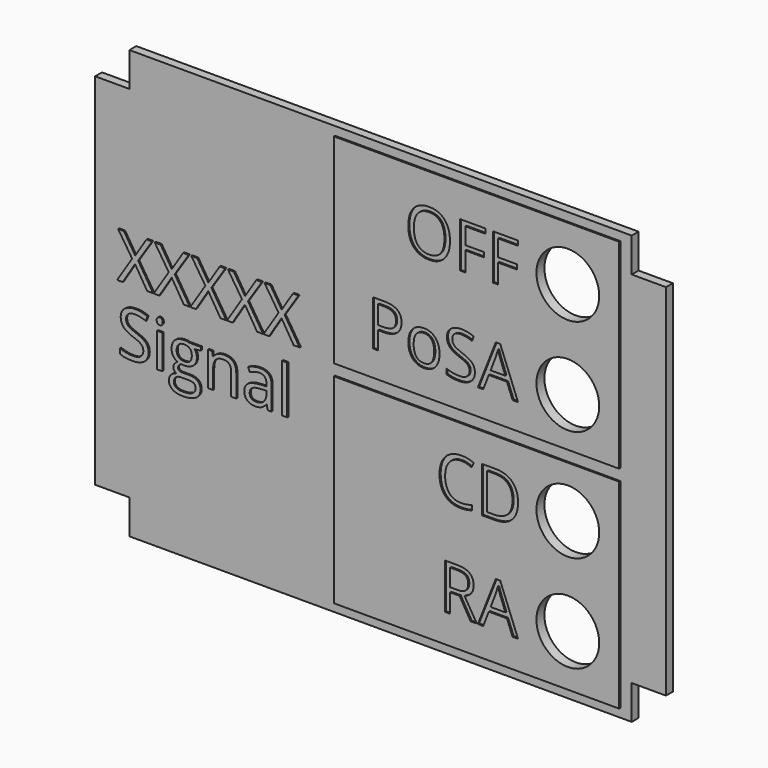
from build123d import *

# Parameters (mm, degrees)
F0_R         = 11
F1_DEPTH     = 3
F2_W         = 100
F2_H         = 70
F2_R         = 11
F2_TEXT_SIZE = 22.2222222222
F3_DEPTH     = 0.5


# Not quite as in the source:
# - Text() gives the source's letters only with a copy of the font that has no kerning and outlines rounded to 1/6400 em; it was checked with that copy


with BuildPart() as f1:
    # F0 (on Front) → F1 (new body)
    with BuildSketch(Plane.XZ):
        Polygon((35.0830127597, 118.6418436468), (-140.9169872403, 118.6418436468), (-140.9169872403, 106.6418436468), (-152.9169872403, 106.6418436468), (-152.9169872403, -19.3581563532), (-140.9169872403, -19.3581563532), (-140.9169872403, -31.3581563532), (35.0830127597, -31.3581563532), (35.0830127597, -19.3581563532), (47.0830127597, -19.3581563532), (47.0830127597, 106.6418436468), (35.0830127597, 106.6418436468), align=None)
        with Locations((13.0830127597, -10.3581563532)):
            Circle(F0_R, mode=Mode.SUBTRACT)
        with Locations((13.0830127597, 23.6418436468)):
            Circle(F0_R, mode=Mode.SUBTRACT)
        with Locations((13.0830127597, 62.6418436468)):
            Circle(F0_R, mode=Mode.SUBTRACT)
        with Locations((13.0830127597, 96.6418436468)):
            Circle(F0_R, mode=Mode.SUBTRACT)
    extrude(amount=F1_DEPTH)

    # F2 (on face) → F3 (join)
    with BuildSketch(Plane.XZ.offset(3)):
        with Locations((-18.9169872403, 6.6418436468)):
            Rectangle(F2_W, F2_H)
        with BuildLine():
            Line((-24.8197650181, -11.760934131), (-28.1322650181, -11.760934131))
            Line((-28.1322650181, -11.760934131), (-28.1322650181, -18.3581563532))
            Line((-28.1322650181, -18.3581563532), (-29.9760150181, -18.3581563532))
            Line((-29.9760150181, -18.3581563532), (-29.9760150181, -2.4935730199))
            Line((-29.9760150181, -2.4935730199), (-25.6253205736, -2.4935730199))
            add(Edge.make_bspline(
                [(-25.6253205736, -2.4935730199), (-22.7051816848, -2.4935730199), (-21.3110844625, -3.6116285755)],
                knots=[0, 0, 0, 1, 1, 1], degree=2))
            add(Edge.make_bspline(
                [(-21.3110844625, -3.6116285755), (-19.9169872403, -4.729684131), (-19.9169872403, -6.9762119088)],
                knots=[0, 0, 0, 1, 1, 1], degree=2))
            add(Edge.make_bspline(
                [(-19.9169872403, -6.9762119088), (-19.9169872403, -10.1220452421), (-23.1079594625, -11.229684131)],
                knots=[0, 0, 0, 1, 1, 1], degree=2))
            Line((-23.1079594625, -11.229684131), (-18.7989316848, -18.3581563532))
            Line((-18.7989316848, -18.3581563532), (-20.9794872403, -18.3581563532))
            Line((-20.9794872403, -18.3581563532), (-24.8197650181, -11.760934131))
        make_face(mode=Mode.SUBTRACT)
        Polygon((-4.3579594625, -18.3581563532), (-6.2676816848, -18.3581563532), (-8.2433761292, -13.3130174643), (-14.6010150181, -13.3130174643), (-16.552403907, -18.3581563532), (-18.4204594625, -18.3581563532), (-12.1496261292, -2.4276007977), (-10.5975427959, -2.4276007977), align=None, mode=Mode.SUBTRACT)
        with Locations((13.0830127597, -10.3581563532)):
            Circle(F2_R, mode=Mode.SUBTRACT)
        with BuildLine():
            add(Edge.make_bspline(
                [(-20.646153907, 29.239065869), (-22.4482372403, 30.082815869), (-24.2503205736, 30.082815869)],
                knots=[0, 0, 0, 1, 1, 1], degree=2))
            add(Edge.make_bspline(
                [(-24.2503205736, 30.082815869), (-26.864903907, 30.082815869), (-28.3787927959, 28.3414964245)],
                knots=[0, 0, 0, 1, 1, 1], degree=2))
            add(Edge.make_bspline(
                [(-28.3787927959, 28.3414964245), (-29.8926816848, 26.6001769801), (-29.8926816848, 23.5723992023)],
                knots=[0, 0, 0, 1, 1, 1], degree=2))
            add(Edge.make_bspline(
                [(-29.8926816848, 23.5723992023), (-29.8926816848, 20.4612880912), (-28.4326122403, 18.7616353134)],
                knots=[0, 0, 0, 1, 1, 1], degree=2))
            add(Edge.make_bspline(
                [(-28.4326122403, 18.7616353134), (-26.9725427959, 17.0619825357), (-24.271153907, 17.0619825357)],
                knots=[0, 0, 0, 1, 1, 1], degree=2))
            add(Edge.make_bspline(
                [(-24.271153907, 17.0619825357), (-22.6114316848, 17.0619825357), (-20.4829594625, 17.6592047579)],
                knots=[0, 0, 0, 1, 1, 1], degree=2))
            Line((-20.4829594625, 17.6592047579), (-20.4829594625, 16.0446214245))
            add(Edge.make_bspline(
                [(-20.4829594625, 16.0446214245), (-22.1322650181, 15.4230936468), (-24.552403907, 15.4230936468)],
                knots=[0, 0, 0, 1, 1, 1], degree=2))
            add(Edge.make_bspline(
                [(-24.552403907, 15.4230936468), (-28.0558761292, 15.4230936468), (-29.9603900181, 17.551565869)],
                knots=[0, 0, 0, 1, 1, 1], degree=2))
            add(Edge.make_bspline(
                [(-29.9603900181, 17.551565869), (-31.864903907, 19.6800380912), (-31.864903907, 23.5967047579)],
                knots=[0, 0, 0, 1, 1, 1], degree=2))
            add(Edge.make_bspline(
                [(-31.864903907, 23.5967047579), (-31.864903907, 26.0480936468), (-30.9482372403, 27.8918436468)],
                knots=[0, 0, 0, 1, 1, 1], degree=2))
            add(Edge.make_bspline(
                [(-30.9482372403, 27.8918436468), (-30.0315705736, 29.7355936468), (-28.3006677959, 30.7338575357)],
                knots=[0, 0, 0, 1, 1, 1], degree=2))
            add(Edge.make_bspline(
                [(-28.3006677959, 30.7338575357), (-26.5697650181, 31.7321214245), (-24.2260150181, 31.7321214245)],
                knots=[0, 0, 0, 1, 1, 1], degree=2))
            add(Edge.make_bspline(
                [(-24.2260150181, 31.7321214245), (-21.7329594625, 31.7321214245), (-19.864903907, 30.8223992023)],
                knots=[0, 0, 0, 1, 1, 1], degree=2))
            Line((-19.864903907, 30.8223992023), (-20.646153907, 29.239065869))
        make_face(mode=Mode.SUBTRACT)
        with BuildLine():
            add(Edge.make_bspline(
                [(-6.4083066848, 29.4560797579), (-4.3579594625, 27.4057325357), (-4.3579594625, 23.7251769801)],
                knots=[0, 0, 0, 1, 1, 1], degree=2))
            add(Edge.make_bspline(
                [(-4.3579594625, 23.7251769801), (-4.3579594625, 19.7980936468), (-6.489903907, 17.7199686468)],
                knots=[0, 0, 0, 1, 1, 1], degree=2))
            add(Edge.make_bspline(
                [(-6.489903907, 17.7199686468), (-8.6218483514, 15.6418436468), (-12.6253205736, 15.6418436468)],
                knots=[0, 0, 0, 1, 1, 1], degree=2))
            Line((-12.6253205736, 15.6418436468), (-17.021153907, 15.6418436468))
            Line((-17.021153907, 15.6418436468), (-17.021153907, 31.5064269801))
            Line((-17.021153907, 31.5064269801), (-12.1600427959, 31.5064269801))
            add(Edge.make_bspline(
                [(-12.1600427959, 31.5064269801), (-8.458653907, 31.5064269801), (-6.4083066848, 29.4560797579)],
                knots=[0, 0, 0, 1, 1, 1], degree=2))
        make_face(mode=Mode.SUBTRACT)
        with Locations((13.0830127597, 23.6418436468)):
            Circle(F2_R, mode=Mode.SUBTRACT)
        with Locations((-18.9169872403, 80.6418436468)):
            Rectangle(F2_W, F2_H)
        with BuildLine():
            add(Edge.make_bspline(
                [(-33.3388622403, 65.0914964245), (-31.8683761292, 63.4300380912), (-31.8683761292, 60.6001769801)],
                knots=[0, 0, 0, 1, 1, 1], degree=2))
            add(Edge.make_bspline(
                [(-31.8683761292, 60.6001769801), (-31.8683761292, 57.6904547579), (-33.3319177959, 56.0567742023)],
                knots=[0, 0, 0, 1, 1, 1], degree=2))
            add(Edge.make_bspline(
                [(-33.3319177959, 56.0567742023), (-34.7954594625, 54.4230936468), (-37.3787927959, 54.4230936468)],
                knots=[0, 0, 0, 1, 1, 1], degree=2))
            add(Edge.make_bspline(
                [(-37.3787927959, 54.4230936468), (-38.9760150181, 54.4230936468), (-40.2121261292, 55.1730936468)],
                knots=[0, 0, 0, 1, 1, 1], degree=2))
            add(Edge.make_bspline(
                [(-40.2121261292, 55.1730936468), (-41.4482372403, 55.9230936468), (-42.1218483514, 57.3223992023)],
                knots=[0, 0, 0, 1, 1, 1], degree=2))
            add(Edge.make_bspline(
                [(-42.1218483514, 57.3223992023), (-42.7954594625, 58.7217047579), (-42.7954594625, 60.6001769801)],
                knots=[0, 0, 0, 1, 1, 1], degree=2))
            add(Edge.make_bspline(
                [(-42.7954594625, 60.6001769801), (-42.7954594625, 63.5064269801), (-41.3405983514, 65.129690869)],
                knots=[0, 0, 0, 1, 1, 1], degree=2))
            add(Edge.make_bspline(
                [(-41.3405983514, 65.129690869), (-39.8857372403, 66.7529547579), (-37.302403907, 66.7529547579)],
                knots=[0, 0, 0, 1, 1, 1], degree=2))
            add(Edge.make_bspline(
                [(-37.302403907, 66.7529547579), (-34.8093483514, 66.7529547579), (-33.3388622403, 65.0914964245)],
                knots=[0, 0, 0, 1, 1, 1], degree=2))
        make_face(mode=Mode.SUBTRACT)
        with BuildLine():
            add(Edge.make_bspline(
                [(-51.1253205736, 70.5064269801), (-45.1808761292, 70.5064269801), (-45.1808761292, 65.8848992023)],
                knots=[0, 0, 0, 1, 1, 1], degree=2))
            add(Edge.make_bspline(
                [(-45.1808761292, 65.8848992023), (-45.1808761292, 63.4751769801), (-46.8249733514, 62.1783019801)],
                knots=[0, 0, 0, 1, 1, 1], degree=2))
            add(Edge.make_bspline(
                [(-46.8249733514, 62.1783019801), (-48.4690705736, 60.8814269801), (-51.5280983514, 60.8814269801)],
                knots=[0, 0, 0, 1, 1, 1], degree=2))
            Line((-51.5280983514, 60.8814269801), (-53.396153907, 60.8814269801))
            Line((-53.396153907, 60.8814269801), (-53.396153907, 54.6418436468))
            Line((-53.396153907, 54.6418436468), (-55.239903907, 54.6418436468))
            Line((-55.239903907, 54.6418436468), (-55.239903907, 70.5064269801))
            Line((-55.239903907, 70.5064269801), (-51.1253205736, 70.5064269801))
        make_face(mode=Mode.SUBTRACT)
        with BuildLine():
            add(Edge.make_bspline(
                [(-20.4239316848, 61.5098992023), (-19.4864316848, 60.489065869), (-19.4864316848, 58.864065869)],
                knots=[0, 0, 0, 1, 1, 1], degree=2))
            add(Edge.make_bspline(
                [(-19.4864316848, 58.864065869), (-19.4864316848, 56.770315869), (-21.005528907, 55.5967047579)],
                knots=[0, 0, 0, 1, 1, 1], degree=2))
            add(Edge.make_bspline(
                [(-21.005528907, 55.5967047579), (-22.5246261292, 54.4230936468), (-25.1287927959, 54.4230936468)],
                knots=[0, 0, 0, 1, 1, 1], degree=2))
            add(Edge.make_bspline(
                [(-25.1287927959, 54.4230936468), (-27.9482372403, 54.4230936468), (-29.4690705736, 55.1522603134)],
                knots=[0, 0, 0, 1, 1, 1], degree=2))
            Line((-29.4690705736, 55.1522603134), (-29.4690705736, 56.9300380912))
            add(Edge.make_bspline(
                [(-29.4690705736, 56.9300380912), (-28.489903907, 56.520315869), (-27.3405983514, 56.2807325357)],
                knots=[0, 0, 0, 1, 1, 1], degree=2))
            add(Edge.make_bspline(
                [(-27.3405983514, 56.2807325357), (-26.1912927959, 56.0411492023), (-25.0628205736, 56.0411492023)],
                knots=[0, 0, 0, 1, 1, 1], degree=2))
            add(Edge.make_bspline(
                [(-25.0628205736, 56.0411492023), (-23.2190705736, 56.0411492023), (-22.2850427959, 56.7408019801)],
                knots=[0, 0, 0, 1, 1, 1], degree=2))
            add(Edge.make_bspline(
                [(-22.2850427959, 56.7408019801), (-21.3510150181, 57.4404547579), (-21.3510150181, 58.6904547579)],
                knots=[0, 0, 0, 1, 1, 1], degree=2))
            add(Edge.make_bspline(
                [(-21.3510150181, 58.6904547579), (-21.3510150181, 59.5133714245), (-21.6826122403, 60.0394130912)],
                knots=[0, 0, 0, 1, 1, 1], degree=2))
            add(Edge.make_bspline(
                [(-21.6826122403, 60.0394130912), (-22.0142094625, 60.5654547579), (-22.7902511292, 61.0116353134)],
                knots=[0, 0, 0, 1, 1, 1], degree=2))
            add(Edge.make_bspline(
                [(-22.7902511292, 61.0116353134), (-23.5662927959, 61.457815869), (-25.1496261292, 62.020315869)],
                knots=[0, 0, 0, 1, 1, 1], degree=2))
            add(Edge.make_bspline(
                [(-25.1496261292, 62.020315869), (-27.3614316848, 62.8119825357), (-28.3110844625, 63.8970519801)],
                knots=[0, 0, 0, 1, 1, 1], degree=2))
            add(Edge.make_bspline(
                [(-28.3110844625, 63.8970519801), (-29.2607372403, 64.9821214245), (-29.2607372403, 66.7286492023)],
                knots=[0, 0, 0, 1, 1, 1], degree=2))
            add(Edge.make_bspline(
                [(-29.2607372403, 66.7286492023), (-29.2607372403, 68.5619825357), (-27.8840011292, 69.6470519801)],
                knots=[0, 0, 0, 1, 1, 1], degree=2))
            add(Edge.make_bspline(
                [(-27.8840011292, 69.6470519801), (-26.5072650181, 70.7321214245), (-24.2364316848, 70.7321214245)],
                knots=[0, 0, 0, 1, 1, 1], degree=2))
            add(Edge.make_bspline(
                [(-24.2364316848, 70.7321214245), (-21.8718483514, 70.7321214245), (-19.8857372403, 69.864065869)],
                knots=[0, 0, 0, 1, 1, 1], degree=2))
            Line((-19.8857372403, 69.864065869), (-20.4621261292, 68.2598992023))
            add(Edge.make_bspline(
                [(-20.4621261292, 68.2598992023), (-22.427403907, 69.082815869), (-24.2815705736, 69.082815869)],
                knots=[0, 0, 0, 1, 1, 1], degree=2))
            add(Edge.make_bspline(
                [(-24.2815705736, 69.082815869), (-25.7468483514, 69.082815869), (-26.5715011292, 68.4543436468)],
                knots=[0, 0, 0, 1, 1, 1], degree=2))
            add(Edge.make_bspline(
                [(-26.5715011292, 68.4543436468), (-27.396153907, 67.8258714245), (-27.396153907, 66.707815869)],
                knots=[0, 0, 0, 1, 1, 1], degree=2))
            add(Edge.make_bspline(
                [(-27.396153907, 66.707815869), (-27.396153907, 65.8848992023), (-27.0923344625, 65.3571214245)],
                knots=[0, 0, 0, 1, 1, 1], degree=2))
            add(Edge.make_bspline(
                [(-27.0923344625, 65.3571214245), (-26.7885150181, 64.8293436468), (-26.0662927959, 64.3901075357)],
                knots=[0, 0, 0, 1, 1, 1], degree=2))
            add(Edge.make_bspline(
                [(-26.0662927959, 64.3901075357), (-25.3440705736, 63.9508714245), (-23.8579594625, 63.4196214245)],
                knots=[0, 0, 0, 1, 1, 1], degree=2))
            add(Edge.make_bspline(
                [(-23.8579594625, 63.4196214245), (-21.3614316848, 62.5307325357), (-20.4239316848, 61.5098992023)],
                knots=[0, 0, 0, 1, 1, 1], degree=2))
        make_face(mode=Mode.SUBTRACT)
        Polygon((-4.3579594625, 54.6418436468), (-6.2676816848, 54.6418436468), (-8.2433761292, 59.6869825357), (-14.6010150181, 59.6869825357), (-16.552403907, 54.6418436468), (-18.4204594625, 54.6418436468), (-12.1496261292, 70.5723992023), (-10.5975427959, 70.5723992023), align=None, mode=Mode.SUBTRACT)
        with Locations((13.0830127597, 62.6418436468)):
            Circle(F2_R, mode=Mode.SUBTRACT)
        with BuildLine():
            add(Edge.make_bspline(
                [(-30.1253205736, 102.5862880912), (-28.2051816848, 100.4161492023), (-28.2051816848, 96.5967047579)],
                knots=[0, 0, 0, 1, 1, 1], degree=2))
            add(Edge.make_bspline(
                [(-28.2051816848, 96.5967047579), (-28.2051816848, 92.7876769801), (-30.1322650181, 90.6053853134)],
                knots=[0, 0, 0, 1, 1, 1], degree=2))
            add(Edge.make_bspline(
                [(-30.1322650181, 90.6053853134), (-32.0593483514, 88.4230936468), (-35.4864316848, 88.4230936468)],
                knots=[0, 0, 0, 1, 1, 1], degree=2))
            add(Edge.make_bspline(
                [(-35.4864316848, 88.4230936468), (-38.989903907, 88.4230936468), (-40.8944177959, 90.567190869)],
                knots=[0, 0, 0, 1, 1, 1], degree=2))
            add(Edge.make_bspline(
                [(-40.8944177959, 90.567190869), (-42.7989316848, 92.7112880912), (-42.7989316848, 96.6175380912)],
                knots=[0, 0, 0, 1, 1, 1], degree=2))
            add(Edge.make_bspline(
                [(-42.7989316848, 96.6175380912), (-42.7989316848, 100.4925380912), (-40.8892094625, 102.6244825357)],
                knots=[0, 0, 0, 1, 1, 1], degree=2))
            add(Edge.make_bspline(
                [(-40.8892094625, 102.6244825357), (-38.9794872403, 104.7564269801), (-35.4655983514, 104.7564269801)],
                knots=[0, 0, 0, 1, 1, 1], degree=2))
            add(Edge.make_bspline(
                [(-35.4655983514, 104.7564269801), (-32.0454594625, 104.7564269801), (-30.1253205736, 102.5862880912)],
                knots=[0, 0, 0, 1, 1, 1], degree=2))
        make_face(mode=Mode.SUBTRACT)
        Polygon((-22.8267094625, 95.4230936468), (-22.8267094625, 88.6418436468), (-24.6704594625, 88.6418436468), (-24.6704594625, 104.5064269801), (-15.8267094625, 104.5064269801), (-15.8267094625, 102.8675380912), (-22.8267094625, 102.8675380912), (-22.8267094625, 97.0619825357), (-16.2503205736, 97.0619825357), (-16.2503205736, 95.4230936468), align=None, mode=Mode.SUBTRACT)
        Polygon((-11.3579594625, 95.4230936468), (-11.3579594625, 88.6418436468), (-13.2017094625, 88.6418436468), (-13.2017094625, 104.5064269801), (-4.3579594625, 104.5064269801), (-4.3579594625, 102.8675380912), (-11.3579594625, 102.8675380912), (-11.3579594625, 97.0619825357), (-4.7815705736, 97.0619825357), (-4.7815705736, 95.4230936468), align=None, mode=Mode.SUBTRACT)
        with Locations((13.0830127597, 96.6418436468)):
            Circle(F2_R, mode=Mode.SUBTRACT)
        with BuildLine():
            add(Edge.make_bspline(
                [(-39.474278907, 101.4404547579), (-40.8475427959, 99.7737880912), (-40.8475427959, 96.5967047579)],
                knots=[0, 0, 0, 1, 1, 1], degree=2))
            add(Edge.make_bspline(
                [(-40.8475427959, 96.5967047579), (-40.8475427959, 93.3744825357), (-39.474278907, 91.707815869)],
                knots=[0, 0, 0, 1, 1, 1], degree=2))
            add(Edge.make_bspline(
                [(-39.474278907, 91.707815869), (-38.1010150181, 90.0411492023), (-35.4864316848, 90.0411492023)],
                knots=[0, 0, 0, 1, 1, 1], degree=2))
            add(Edge.make_bspline(
                [(-35.4864316848, 90.0411492023), (-32.8510150181, 90.0411492023), (-31.505528907, 91.7008714245)],
                knots=[0, 0, 0, 1, 1, 1], degree=2))
            add(Edge.make_bspline(
                [(-31.505528907, 91.7008714245), (-30.1600427959, 93.3605936468), (-30.1600427959, 96.5967047579)],
                knots=[0, 0, 0, 1, 1, 1], degree=2))
            add(Edge.make_bspline(
                [(-30.1600427959, 96.5967047579), (-30.1600427959, 99.7980936468), (-31.5003205736, 101.4526075357)],
                knots=[0, 0, 0, 1, 1, 1], degree=2))
            add(Edge.make_bspline(
                [(-31.5003205736, 101.4526075357), (-32.8405983514, 103.1071214245), (-35.4655983514, 103.1071214245)],
                knots=[0, 0, 0, 1, 1, 1], degree=2))
            add(Edge.make_bspline(
                [(-35.4655983514, 103.1071214245), (-38.1010150181, 103.1071214245), (-39.474278907, 101.4404547579)],
                knots=[0, 0, 0, 1, 1, 1], degree=2))
        make_face()
        with BuildLine():
            add(Edge.make_bspline(
                [(-7.9708066848, 18.8588575357), (-6.3093483514, 20.4821214245), (-6.3093483514, 23.6592047579)],
                knots=[0, 0, 0, 1, 1, 1], degree=2))
            add(Edge.make_bspline(
                [(-6.3093483514, 23.6592047579), (-6.3093483514, 26.7633714245), (-7.8666400181, 28.3362880912)],
                knots=[0, 0, 0, 1, 1, 1], degree=2))
            add(Edge.make_bspline(
                [(-7.8666400181, 28.3362880912), (-9.4239316848, 29.9092047579), (-12.4968483514, 29.9092047579)],
                knots=[0, 0, 0, 1, 1, 1], degree=2))
            Line((-12.4968483514, 29.9092047579), (-15.177403907, 29.9092047579))
            Line((-15.177403907, 29.9092047579), (-15.177403907, 17.2355936468))
            Line((-15.177403907, 17.2355936468), (-12.9308761292, 17.2355936468))
            add(Edge.make_bspline(
                [(-12.9308761292, 17.2355936468), (-9.6322650181, 17.2355936468), (-7.9708066848, 18.8588575357)],
                knots=[0, 0, 0, 1, 1, 1], degree=2))
        make_face()
        with Locations((-144.9169872403, 46.6418436468)):
            Text('XXXXX', F2_TEXT_SIZE, font='Open Sans', text_align=(TextAlign.LEFT, TextAlign.BOTTOM))
        with BuildLine():
            add(Edge.make_bspline(
                [(-40.0263622403, 64.0602464245), (-40.927403907, 62.8987880912), (-40.927403907, 60.6001769801)],
                knots=[0, 0, 0, 1, 1, 1], degree=2))
            add(Edge.make_bspline(
                [(-40.927403907, 60.6001769801), (-40.927403907, 58.3189269801), (-40.0159455736, 57.1262186468)],
                knots=[0, 0, 0, 1, 1, 1], degree=2))
            add(Edge.make_bspline(
                [(-40.0159455736, 57.1262186468), (-39.1044872403, 55.9335103134), (-37.3371261292, 55.9335103134)],
                knots=[0, 0, 0, 1, 1, 1], degree=2))
            add(Edge.make_bspline(
                [(-37.3371261292, 55.9335103134), (-35.5662927959, 55.9335103134), (-34.6496261292, 57.1210103134)],
                knots=[0, 0, 0, 1, 1, 1], degree=2))
            add(Edge.make_bspline(
                [(-34.6496261292, 57.1210103134), (-33.7329594625, 58.3085103134), (-33.7329594625, 60.6001769801)],
                knots=[0, 0, 0, 1, 1, 1], degree=2))
            add(Edge.make_bspline(
                [(-33.7329594625, 60.6001769801), (-33.7329594625, 62.8675380912), (-34.6496261292, 64.0446214245)],
                knots=[0, 0, 0, 1, 1, 1], degree=2))
            add(Edge.make_bspline(
                [(-34.6496261292, 64.0446214245), (-35.5662927959, 65.2217047579), (-37.3579594625, 65.2217047579)],
                knots=[0, 0, 0, 1, 1, 1], degree=2))
            add(Edge.make_bspline(
                [(-37.3579594625, 65.2217047579), (-39.1253205736, 65.2217047579), (-40.0263622403, 64.0602464245)],
                knots=[0, 0, 0, 1, 1, 1], degree=2))
        make_face()
        with BuildLine():
            Line((-53.396153907, 68.9092047579), (-53.396153907, 62.4647603134))
            Line((-53.396153907, 62.4647603134), (-51.7329594625, 62.4647603134))
            add(Edge.make_bspline(
                [(-51.7329594625, 62.4647603134), (-49.2815705736, 62.4647603134), (-48.1860844625, 63.2564269801)],
                knots=[0, 0, 0, 1, 1, 1], degree=2))
            add(Edge.make_bspline(
                [(-48.1860844625, 63.2564269801), (-47.0905983514, 64.0480936468), (-47.0905983514, 65.7980936468)],
                knots=[0, 0, 0, 1, 1, 1], degree=2))
            add(Edge.make_bspline(
                [(-47.0905983514, 65.7980936468), (-47.0905983514, 67.3710103134), (-48.1218483514, 68.1401075357)],
                knots=[0, 0, 0, 1, 1, 1], degree=2))
            add(Edge.make_bspline(
                [(-48.1218483514, 68.1401075357), (-49.1530983514, 68.9092047579), (-51.333653907, 68.9092047579)],
                knots=[0, 0, 0, 1, 1, 1], degree=2))
            Line((-51.333653907, 68.9092047579), (-53.396153907, 68.9092047579))
        make_face()
        with BuildLine():
            Line((-28.1322650181, -4.1116285755), (-28.1322650181, -10.1776007977))
            Line((-28.1322650181, -10.1776007977), (-25.6010150181, -10.1776007977))
            add(Edge.make_bspline(
                [(-25.6010150181, -10.1776007977), (-23.6496261292, -10.1776007977), (-22.7381677959, -9.401559131)],
                knots=[0, 0, 0, 1, 1, 1], degree=2))
            add(Edge.make_bspline(
                [(-22.7381677959, -9.401559131), (-21.8267094625, -8.6255174643), (-21.8267094625, -7.073434131)],
                knots=[0, 0, 0, 1, 1, 1], degree=2))
            add(Edge.make_bspline(
                [(-21.8267094625, -7.073434131), (-21.8267094625, -5.5005174643), (-22.7537927959, -4.8060730199)],
                knots=[0, 0, 0, 1, 1, 1], degree=2))
            add(Edge.make_bspline(
                [(-22.7537927959, -4.8060730199), (-23.6808761292, -4.1116285755), (-25.7329594625, -4.1116285755)],
                knots=[0, 0, 0, 1, 1, 1], degree=2))
            Line((-25.7329594625, -4.1116285755), (-28.1322650181, -4.1116285755))
        make_face()
        with BuildLine():
            Line((-13.9482372403, 61.3467047579), (-8.8162927959, 61.3467047579))
            Line((-8.8162927959, 61.3467047579), (-10.6635150181, 66.2633714245))
            add(Edge.make_bspline(
                [(-10.6635150181, 66.2633714245), (-11.021153907, 67.1973992023), (-11.3996261292, 68.551565869)],
                knots=[0, 0, 0, 1, 1, 1], degree=2))
            add(Edge.make_bspline(
                [(-11.3996261292, 68.551565869), (-11.6392094625, 67.5098992023), (-12.083653907, 66.2633714245)],
                knots=[0, 0, 0, 1, 1, 1], degree=2))
            Line((-12.083653907, 66.2633714245), (-13.9482372403, 61.3467047579))
        make_face()
        with BuildLine():
            Line((-13.9482372403, -11.6532952421), (-8.8162927959, -11.6532952421))
            Line((-8.8162927959, -11.6532952421), (-10.6635150181, -6.7366285755))
            add(Edge.make_bspline(
                [(-10.6635150181, -6.7366285755), (-11.021153907, -5.8026007977), (-11.3996261292, -4.448434131)],
                knots=[0, 0, 0, 1, 1, 1], degree=2))
            add(Edge.make_bspline(
                [(-11.3996261292, -4.448434131), (-11.6392094625, -5.4901007977), (-12.083653907, -6.7366285755)],
                knots=[0, 0, 0, 1, 1, 1], degree=2))
            Line((-12.083653907, -6.7366285755), (-13.9482372403, -11.6532952421))
        make_face()
        with Locations((-144.9169872403, 23.6418436468)):
            Text('Signal', F2_TEXT_SIZE, font='Open Sans', text_align=(TextAlign.LEFT, TextAlign.BOTTOM))
    extrude(amount=F3_DEPTH)


solid = f1.part
